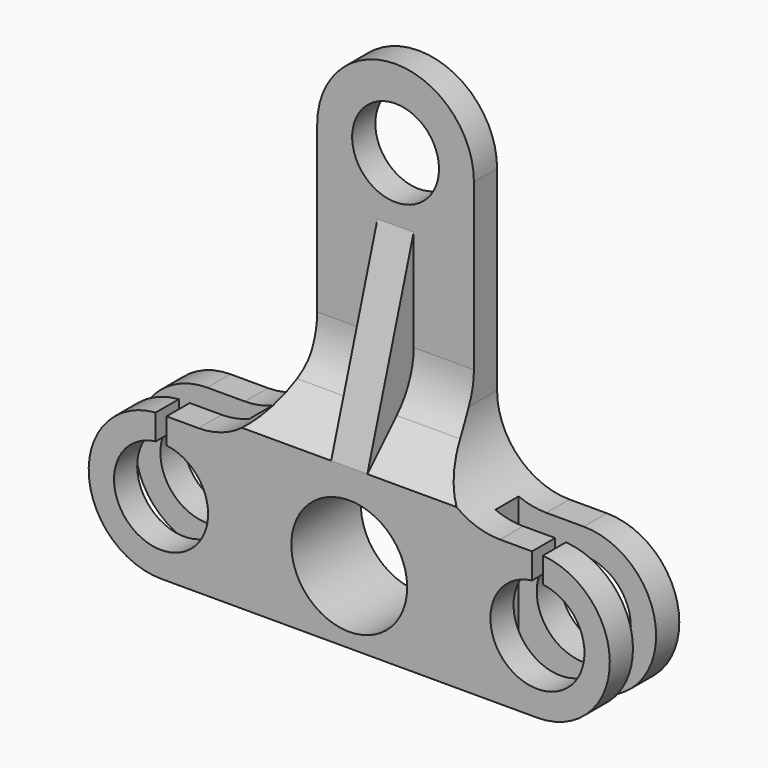
from build123d import *

# Parameters (mm, degrees)
F0_R     = 3.25
F0_R_2   = 4
F0_R_3   = 3
F1_DEPTH = 3
F3_DEPTH = 12.5
F5_DEPTH = 1.25
F6_W     = 9.5
F6_H     = 2
F7_DEPTH = 12.5
F8_W     = 0.75
F8_H     = 4
F9_DEPTH = 2


# Not quite as in the source:
# - a pattern or mirror of a feature is missing from the dataset's text; its kind, count and spacing are read off the source's solid


with BuildPart() as f1:
    # F0 (on Front) → F1 (new body, symmetric)
    with BuildSketch(Plane.XZ):
        with BuildLine():
            Line((-13, -5), (13, -5))
            ThreePointArc((13, -5), (18, 0), (13, 5))
            Line((13, 5), (10.4125417955, 5))
            ThreePointArc((10.4125417955, 5), (6.8770078896, 6.4644660941), (5.4125417955, 10))
            Line((5.4125417955, 10), (5.4125417955, 6))
            Line((5.4125417955, 6), (-5.4125417955, 6))
            Line((-5.4125417955, 6), (-5.4125417955, 10))
            ThreePointArc((-5.4125417955, 10), (-6.8770078896, 6.4644660941), (-10.4125417955, 5))
            Line((-10.4125417955, 5), (-13, 5))
            ThreePointArc((-13, 5), (-18, 0), (-13, -5))
        make_face()
        with Locations((-13, 0)):
            Circle(F0_R, mode=Mode.SUBTRACT)
        Circle(F0_R_2, mode=Mode.SUBTRACT)
        with Locations((13, 0)):
            Circle(F0_R, mode=Mode.SUBTRACT)
        with BuildLine():
            Line((5.4125417955, 6), (5.4125417955, 10))
            Line((5.4125417955, 10), (5.4125417955, 23.5))
            ThreePointArc((5.4125417955, 23.5), (0, 28.9125417955), (-5.4125417955, 23.5))
            Line((-5.4125417955, 23.5), (-5.4125417955, 10))
            Line((-5.4125417955, 10), (-5.4125417955, 6))
            Line((-5.4125417955, 6), (5.4125417955, 6))
        make_face()
        with Locations((0, 23.5)):
            Circle(F0_R_3, mode=Mode.SUBTRACT)
    extrude(amount=F1_DEPTH, both=True)

    # F2 (on Right) → F3 (cut, symmetric)
    with BuildSketch(Plane.YZ):
        with BuildLine():
            Line((1, 28.9125417955), (-3, 28.9125417955))
            Line((-3, 28.9125417955), (-3, 23.5))
            Line((-3, 23.5), (-3, 10))
            Line((-3, 10), (-3, 6))
            Line((-3, 6), (-0.4644660941, 8.5355339059))
            ThreePointArc((-0.4644660941, 8.5355339059), (0.6193976626, 10.15765065), (1, 12.0710678119))
            Line((1, 12.0710678119), (1, 28.9125417955))
        make_face()
    extrude(amount=F3_DEPTH, both=True, mode=Mode.SUBTRACT)

    # F4 (on Right) → F5 (join, symmetric)
    with BuildSketch(Plane.YZ):
        Polygon((1, 19.0834104739), (-3, 6), (1.3459398516, 6), (1.3459398516, 20.2149287434), align=None)
    extrude(amount=F5_DEPTH, both=True)

    # F6 (on Top) → F7 (cut, symmetric)
    with BuildSketch(Plane.XY):
        with Locations((13.25, 0)):
            Rectangle(F6_W, F6_H)
    f7 = extrude(amount=F7_DEPTH, both=True, mode=Mode.SUBTRACT)

    # F7_copies: F7 across plane
    add(f7.mirror(Plane(origin=(0, 0, 0), x_dir=(0, 0, -1), z_dir=(-1, 0, 0))), mode=Mode.SUBTRACT)

    # F8 (on face) → F9 (cut)
    with BuildSketch(Plane.XZ.offset(3)):
        with Locations((13, 5)):
            Rectangle(F8_W, F8_H)
    f9 = extrude(amount=-F9_DEPTH, mode=Mode.SUBTRACT)

    # F9_copies: F9 across plane
    add(f9.mirror(Plane(origin=(0, 0, 0), x_dir=(0, 0, -1), z_dir=(-1, 0, 0))), mode=Mode.SUBTRACT)


solid = f1.part
